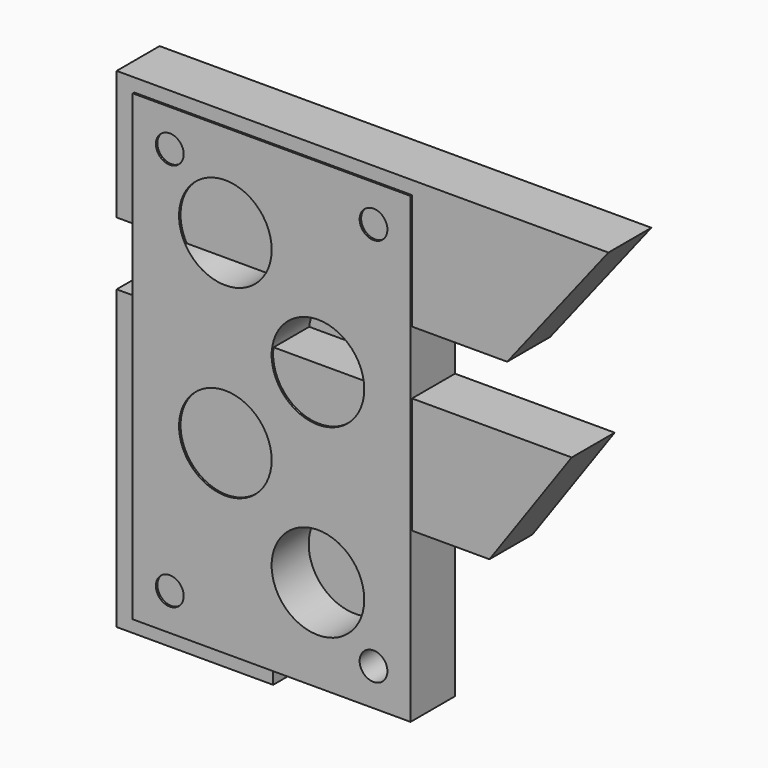
from build123d import *

# Parameters (mm, degrees)
F1_DEPTH = 7.366
F3_W     = 38.1
F3_H     = 63.5
F4_DEPTH = 7.62
F5_R     = 6.35
F5_R_2   = 1.905
F6_DEPTH = 6.35
F2_R     = 6.35
F2_R_2   = 1.905
F7_DEPTH = 6.35


# Not quite as in the source:
# - a feature of the source that left no trace in its solid (it failed there, or was rolled back) is left out


with BuildPart() as f1:
    # F0 (on Front) → F1 (new body)
    with BuildSketch(Plane.XZ):
        Polygon((40.94883606, 7.20073871), (-21.4626698, 7.20073871), (-21.4626698, -33.57456201), (0, -33.57456201), (0, -8.76236119), (29.67054772, -8.76236119), align=None)
    extrude(amount=F1_DEPTH)


with BuildPart() as f1b:
    # F0 (on Front) → F1, piece 2 (new body)
    with BuildSketch(Plane.XZ):
        Polygon((-21.4626698, 15.87636017), (32.0997072, 15.87636017), (45.98066242, 33.57456201), (-21.4626698, 33.57456201), align=None)
    extrude(amount=F1_DEPTH)


with BuildPart() as f4:
    # F3 (on Front) → F4 (new body)
    with BuildSketch(Plane.XZ):
        Rectangle(F3_W, F3_H)
    extrude(amount=F4_DEPTH)

    # F5 (on face) → F6 (cut)
    with BuildSketch(Plane.XZ.offset(7.62)):
        with Locations((-6.35, 19.05)):
            Circle(F5_R)
        with Locations((6.35, 6.35)):
            Circle(F5_R)
        with Locations((-6.35, -6.35)):
            Circle(F5_R)
        with Locations((6.35, -19.05)):
            Circle(F5_R)
        with Locations((13.97, 26.67)):
            Circle(F5_R_2)
        with Locations((13.97, -26.67)):
            Circle(F5_R_2)
        with Locations((-13.97, -26.67)):
            Circle(F5_R_2)
        with Locations((-13.97, 26.67)):
            Circle(F5_R_2)
    extrude(amount=-F6_DEPTH, mode=Mode.SUBTRACT)


with BuildPart() as f7_tool:
    # F2 (on face) → F7 (new body)
    with BuildSketch(Plane.XZ):
        with Locations((-8.89, 24.72546109)):
            Circle(F2_R)
        with Locations((8.89, 24.72546109)):
            Circle(F2_R)
        with Locations((8.89, -0.78081124)):
            Circle(F2_R)
        with Locations((-8.89, -0.78081124)):
            Circle(F2_R)
        with Locations((-8.89, -22.9579730041)):
            Circle(F2_R)
        with Locations((32.69018481, 24.72546109)):
            Circle(F2_R_2)
        with Locations((-17.6526698, 29.76456201)):
            Circle(F2_R_2)
        with Locations((-17.6526698, 19.68636017)):
            Circle(F2_R_2)
        with Locations((28.95969189, -0.78081124)):
            Circle(F2_R_2)
        with Locations((-17.6526698, 3.39073871)):
            Circle(F2_R_2)
        with Locations((-17.6526698, -29.76456201)):
            Circle(F2_R_2)
    extrude(amount=F7_DEPTH)


with BuildPart() as f1_1:
    add(f1.part)

    # F7: cut by f7_tool
    add(f7_tool.part, mode=Mode.SUBTRACT)


with BuildPart() as f1b_1:
    add(f1b.part)

    # F7: cut by f7_tool
    add(f7_tool.part, mode=Mode.SUBTRACT)


solid = Compound([f4.part, f1_1.part, f1b_1.part])
